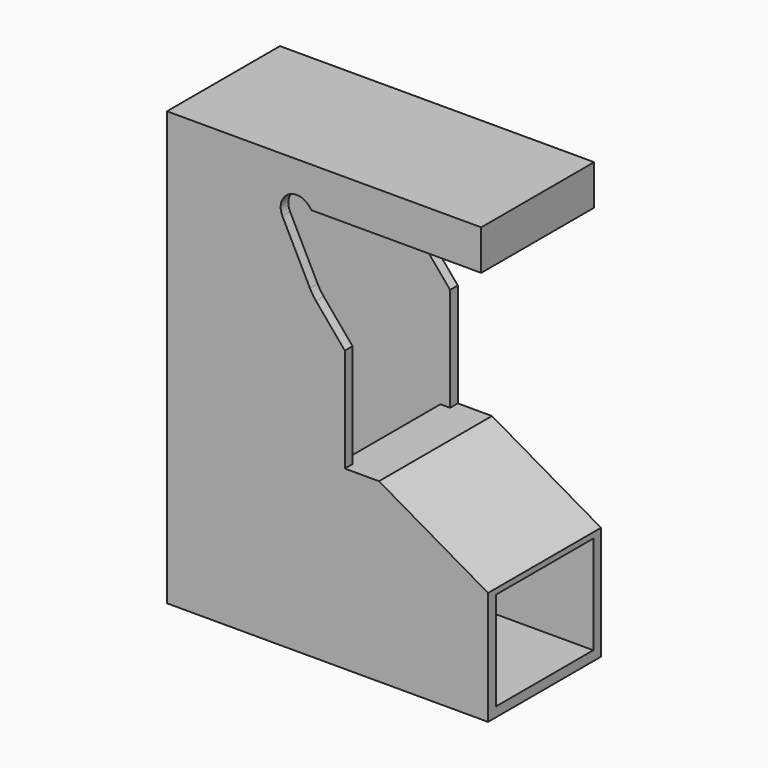
from build123d import *

# Parameters (mm, degrees)
F0_R         = 2.3
F1_DEPTH     = 8.8
F2_T         = -1.2
F3_DEPTH     = 1.2
F4_DEPTH     = 28.2
F5_DEPTH     = 1.2
F6_W         = 23
F6_H         = 2.2
F7_DEPTH     = 1.2
F9_DEPTH     = 17.6
F10_W        = 15.2
F10_H        = 3.8
F11_DEPTH    = 25
F12_T4_DEPTH = 15.2


# Not quite as in the source:
# - a fillet or chamfer that OpenCascade refuses, or shapes differently, is made with other operations: its cross-section is extruded or revolved along the edge and cut away or added
# - a feature names something its author has since deleted; it is built from what else it names


with BuildPart() as f1:
    # F0 (on Front) → F1 (new body, symmetric)
    with BuildSketch(Plane.XZ):
        Polygon((-40.0227420032, 54), (-40.0227420032, 0), (0, 0), (0, 14.1528282114), (-13.5917002335, 22), (-17.8529980872, 22), (-17.8529980872, 49), (-0.8529980872, 49), (-0.8529980872, 54), (-17.8529980872, 54), align=None)
        with Locations((-24.1529980872, 48.7)):
            Circle(F0_R, mode=Mode.SUBTRACT)
        with Locations((-24.1529980872, 48.7)):
            Circle(F0_R)
    extrude(amount=F1_DEPTH, both=True)

    # F2
    f2_openings = [f1.faces().sort_by_distance(p)[0] for p in [
        (-40.022742, 0, 27),
    ]]
    offset(amount=F2_T, openings=f2_openings, kind=Kind.INTERSECTION)

    # F3 (cut, through all): a face of the model
    f3_faces = [f1.faces().sort_by_distance(p)[0] for p in [
        (-2.0529980872, 0, 51.5),
    ]]
    extrude(f3_faces, amount=-F3_DEPTH, mode=Mode.SUBTRACT)

    # F4 (cut, through all): a face of the model
    f4_faces = [f1.faces().sort_by_distance(p)[0] for p in [
        (-9.9529980872, 0, 50.2),
    ]]
    extrude(f4_faces, amount=-F4_DEPTH, mode=Mode.SUBTRACT)

    # F5 (cut, through all): a face of the model
    f5_faces = [f1.faces().sort_by_distance(p)[0] for p in [
        (-1.2, 0, 7.3300039442),
    ]]
    extrude(f5_faces, amount=-F5_DEPTH, mode=Mode.SUBTRACT)

    # F6 (on face) → F7 (cut, through all)
    with BuildSketch(Plane(origin=(0, 0, 0), x_dir=(1, 0, 0), z_dir=(0, 0, -1))):
        with Locations((-28.5227420032, 0)):
            Rectangle(F6_W, F6_H)
    extrude(amount=-F7_DEPTH, mode=Mode.SUBTRACT)

    # F8 (on face) → F9 (cut, through all)
    with BuildSketch(Plane.XZ.offset(8.8)):
        with BuildLine():
            ThreePointArc((-22.2107439409, 40.3830760217), (-22.207256, 45.7916724587), (-17.8529980872, 49))
            Line((-17.8529980872, 49), (-21.9990858511, 49))
            Line((-21.9990858511, 49), (-22.3439980513, 49.3965202671))
            ThreePointArc((-22.3439980513, 49.3965202671), (-24.9680683048, 49.7442269385), (-25.6389133718, 47.1836388185))
            Line((-25.6389133718, 47.1836388185), (-22.2107439409, 40.3830760217))
        make_face()
        with BuildLine():
            Line((-17.8529980872, 34.9413308483), (-17.8529980872, 49))
            ThreePointArc((-17.8529980872, 49), (-22.207256, 45.7916724587), (-22.2107439409, 40.3830760217))
            ThreePointArc((-22.2107439409, 40.3830760217), (-21.8634478438, 39.783103161), (-21.4492647459, 39.2271945588))
            Line((-21.4492647459, 39.2271945588), (-17.8529980872, 34.9413308483))
        make_face()
    extrude(amount=-F9_DEPTH, mode=Mode.SUBTRACT)

    # F10 (on face) → F11 (join)
    with BuildSketch(Plane.YZ.offset(-0.8529980872)):
        with Locations((0, 50.9)):
            Rectangle(F10_W, F10_H)
    extrude(amount=-F11_DEPTH)

    # F12: chamfer of 9 x 5.1961524227 on 1 edges, made by hand


with BuildPart() as f12_tool2:
    # F12_s3 → F12_t4 (new body)
    with BuildSketch(Plane.XZ.offset(7.6)):
        Polygon((-16.8529980872, 49), (-25.8529980872, 54.1961524227), (-25.8529980872, 49), align=None)
    extrude(amount=-F12_T4_DEPTH)

    split(bisect_by=Plane.XY.offset(52.8), keep=Keep.BOTTOM)


with BuildPart() as f1_1:
    add(f1.part)

    # F12_t1: cut F12_tool2
    add(f12_tool2.part, mode=Mode.SUBTRACT)


solid = f1_1.part
